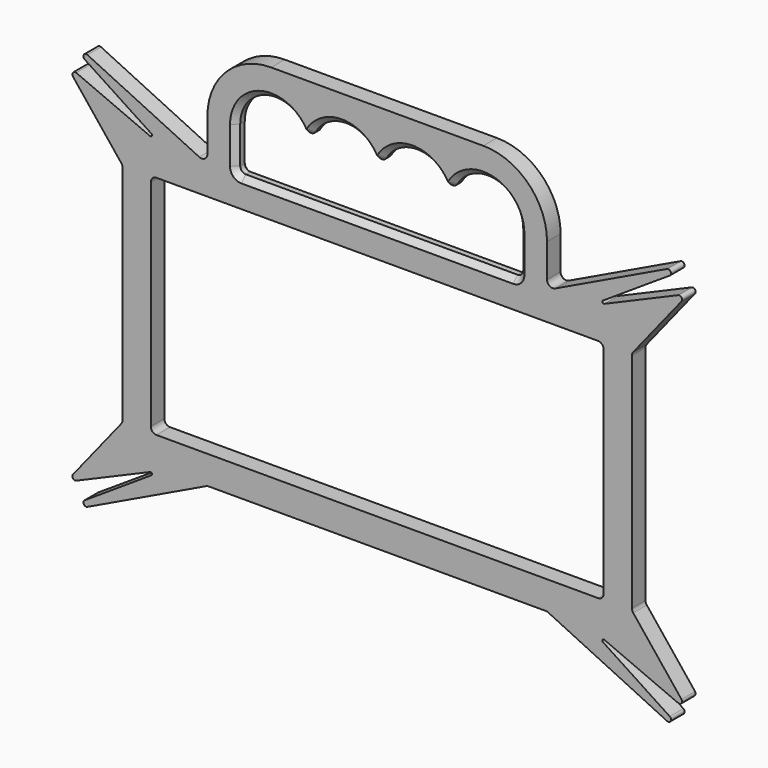
from build123d import *

# Parameters (mm, degrees)
F1_DEPTH = 6
F2_SIZE  = 1.99999


# Not quite as in the source:
# - a fillet or chamfer is up to 0.001 mm smaller than in the source, because OpenCascade refuses the exact size


with BuildPart() as f1:
    # F0 (on Front) → F1 (new body)
    with BuildSketch(Plane.XZ):
        with BuildLine():
            Line((-59.5457699822, -50), (59.5457699822, -50))
            ThreePointArc((59.5457699822, -50), (59.9887196894, -50.0496678342), (60.409669044, -50.1962044431))
            Line((60.409669044, -50.1962044431), (102.3891955872, -70.3016279512))
            ThreePointArc((102.3891955872, -70.3016279512), (103.6924020371, -69.8905574143), (103.3686877569, -68.5629523894))
            Line((103.3686877569, -68.5629523894), (79.7822069148, -53.1292204996))
            ThreePointArc((79.7822069148, -53.1292204996), (79.6153206959, -52.4745670657), (80.2529378835, -52.2512590929))
            Line((80.2529378835, -52.2512590929), (106.3328214803, -63.428352063))
            ThreePointArc((106.3328214803, -63.428352063), (107.5225378807, -63.1147703845), (107.5076095883, -61.8845119854))
            Line((107.5076095883, -61.8845119854), (90.4382623811, -40.5478279764))
            ThreePointArc((90.4382623811, -40.5478279764), (90.1127433617, -39.9604517642), (90, -39.2984378813))
            Line((90, -39.2984378813), (90, 39.2984378813))
            ThreePointArc((90, 39.2984378813), (90.1127433617, 39.9604517642), (90.4382623811, 40.5478279764))
            Line((90.4382623811, 40.5478279764), (107.5076095883, 61.8845119854))
            ThreePointArc((107.5076095883, 61.8845119854), (107.5225378807, 63.1147703845), (106.3328214803, 63.428352063))
            Line((106.3328214803, 63.428352063), (80.2529378835, 52.2512590929))
            ThreePointArc((80.2529378835, 52.2512590929), (79.6153206959, 52.4745670657), (79.7822069148, 53.1292204996))
            Line((79.7822069148, 53.1292204996), (103.3686877569, 68.5629523894))
            ThreePointArc((103.3686877569, 68.5629523894), (103.6924020371, 69.8905574143), (102.3891955872, 70.3016279512))
            Line((102.3891955872, 70.3016279512), (62.8638990618, 51.3716186976))
            ThreePointArc((62.8638990618, 51.3716186976), (60.9341196417, 51.4831084128), (60, 53.1754142545))
            Line((60, 53.1754142545), (60, 65))
            ThreePointArc((60, 65), (53.4099025767, 80.9099025767), (37.5, 87.5))
            Line((37.5, 87.5), (0, 87.5))
            Line((0, 87.5), (-37.5, 87.5))
            ThreePointArc((-37.5, 87.5), (-53.4099025767, 80.9099025767), (-60, 65))
            Line((-60, 65), (-60, 53.1754142545))
            ThreePointArc((-60, 53.1754142545), (-60.9341196417, 51.4831084128), (-62.8638990618, 51.3716186976))
            Line((-62.8638990618, 51.3716186976), (-102.3891955872, 70.3016279512))
            ThreePointArc((-102.3891955872, 70.3016279512), (-103.6924020371, 69.8905574143), (-103.3686877569, 68.5629523894))
            Line((-103.3686877569, 68.5629523894), (-79.7822069148, 53.1292204996))
            ThreePointArc((-79.7822069148, 53.1292204996), (-79.6153206959, 52.4745670657), (-80.2529378835, 52.2512590929))
            Line((-80.2529378835, 52.2512590929), (-106.3328214803, 63.428352063))
            ThreePointArc((-106.3328214803, 63.428352063), (-107.5225378807, 63.1147703845), (-107.5076095883, 61.8845119854))
            Line((-107.5076095883, 61.8845119854), (-90.4382623811, 40.5478279764))
            ThreePointArc((-90.4382623811, 40.5478279764), (-90.1127433617, 39.9604517642), (-90, 39.2984378813))
            Line((-90, 39.2984378813), (-90, -39.2984378813))
            ThreePointArc((-90, -39.2984378813), (-90.1127433617, -39.9604517642), (-90.4382623811, -40.5478279764))
            Line((-90.4382623811, -40.5478279764), (-107.5076095883, -61.8845119854))
            ThreePointArc((-107.5076095883, -61.8845119854), (-107.5225378807, -63.1147703845), (-106.3328214803, -63.428352063))
            Line((-106.3328214803, -63.428352063), (-80.2529378835, -52.2512590929))
            ThreePointArc((-80.2529378835, -52.2512590929), (-79.6153206959, -52.4745670657), (-79.7822069148, -53.1292204996))
            Line((-79.7822069148, -53.1292204996), (-103.3686877569, -68.5629523894))
            ThreePointArc((-103.3686877569, -68.5629523894), (-103.6924020371, -69.8905574143), (-102.3891955872, -70.3016279512))
            Line((-102.3891955872, -70.3016279512), (-60.409669044, -50.1962044431))
            ThreePointArc((-60.409669044, -50.1962044431), (-59.9887196894, -50.0496678342), (-59.5457699822, -50))
        make_face()
        with BuildLine():
            Line((-78, 40), (78, 40))
            ThreePointArc((78, 40), (79.4142135624, 39.4142135624), (80, 38))
            Line((80, 38), (80, -38))
            ThreePointArc((80, -38), (79.4142135624, -39.4142135624), (78, -40))
            Line((78, -40), (-78, -40))
            ThreePointArc((-78, -40), (-79.4142135624, -39.4142135624), (-80, -38))
            Line((-80, -38), (-80, 38))
            ThreePointArc((-80, 38), (-79.4142135624, 39.4142135624), (-78, 40))
        make_face(mode=Mode.SUBTRACT)
        with BuildLine():
            Line((48, 50), (40, 50))
            Line((40, 50), (0, 50))
            Line((0, 50), (-25, 50))
            Line((-25, 50), (-40, 50))
            Line((-40, 50), (-48, 50))
            ThreePointArc((-48, 50), (-49.4142135624, 50.5857864376), (-50, 52))
            Line((-50, 52), (-50, 65))
            ThreePointArc((-50, 65), (-40.7826608215, 77.0612660169), (-26.724137931, 71.3348872658))
            ThreePointArc((-26.724137931, 71.3348872658), (-25, 70.3484692283), (-23.275862069, 71.3348872658))
            ThreePointArc((-23.275862069, 71.3348872658), (-12.5, 77.5), (-1.724137931, 71.3348872658))
            ThreePointArc((-1.724137931, 71.3348872658), (0, 70.3484692283), (1.724137931, 71.3348872658))
            ThreePointArc((1.724137931, 71.3348872658), (12.5, 77.5), (23.275862069, 71.3348872658))
            ThreePointArc((23.275862069, 71.3348872658), (25, 70.3484692283), (26.724137931, 71.3348872658))
            ThreePointArc((26.724137931, 71.3348872658), (40.7826608215, 77.0612660169), (50, 65))
            Line((50, 65), (50, 52))
            ThreePointArc((50, 52), (49.4142135624, 50.5857864376), (48, 50))
        make_face(mode=Mode.SUBTRACT)
    extrude(amount=F1_DEPTH)

    # F2 (size 2 in the source; OpenCascade refuses exactly that, so slightly less here)
    f2_edges = [f1.edges().sort_by_distance(p)[0] for p in [
        (0, -6, 50),
        (0, 0, 50),
    ]]
    chamfer(f2_edges, length=F2_SIZE)


solid = f1.part
